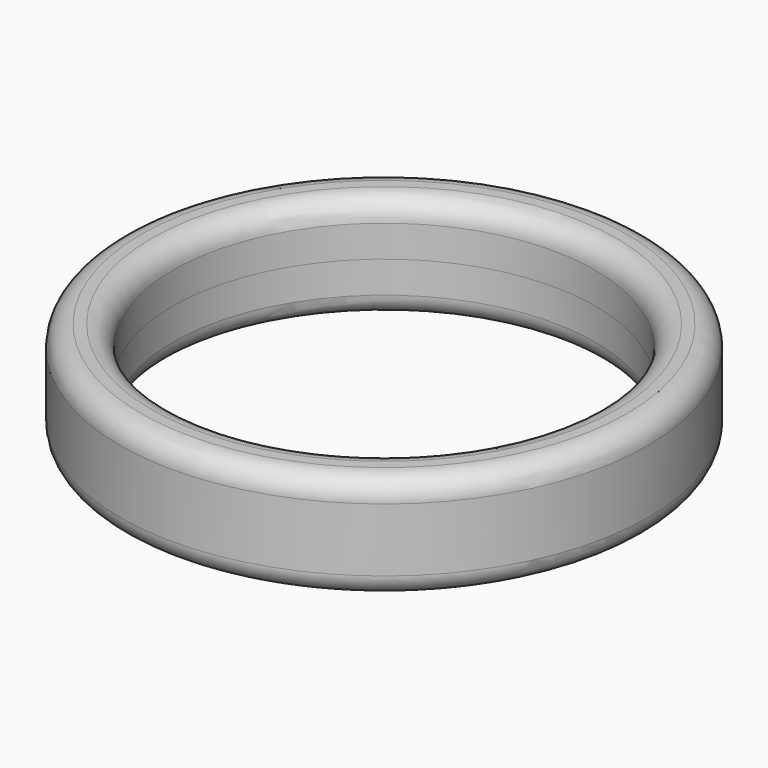
from build123d import *

# Parameters (mm, degrees)
F0_R          = 12.7
F0_R_2        = 10.16
F1_DEPTH      = 2.54
F1_DEPTH_BACK = 2.54
F2_R          = 1.016


with BuildPart() as f1:
    # F0 (on Top) → F1 (new body, two sides)
    with BuildSketch(Plane.XY) as f1_sk:
        Circle(F0_R)
        Circle(F0_R_2, mode=Mode.SUBTRACT)
    extrude(amount=F1_DEPTH)
    extrude(f1_sk.sketch, amount=-F1_DEPTH_BACK)

    # F2
    f2_edges = [f1.edges().sort_by_distance(p)[0] for p in [
        (12.7, 0, -1.27),
        (-12.7, 0, 0),
        (-12.7, 0, -2.54),
        (10.16, 0, -1.27),
        (-10.16, 0, 0),
        (-10.16, 0, -2.54),
        (-12.7, 0, 2.54),
        (-10.16, 0, 2.54),
    ]]
    fillet(f2_edges, radius=F2_R)


solid = f1.part
